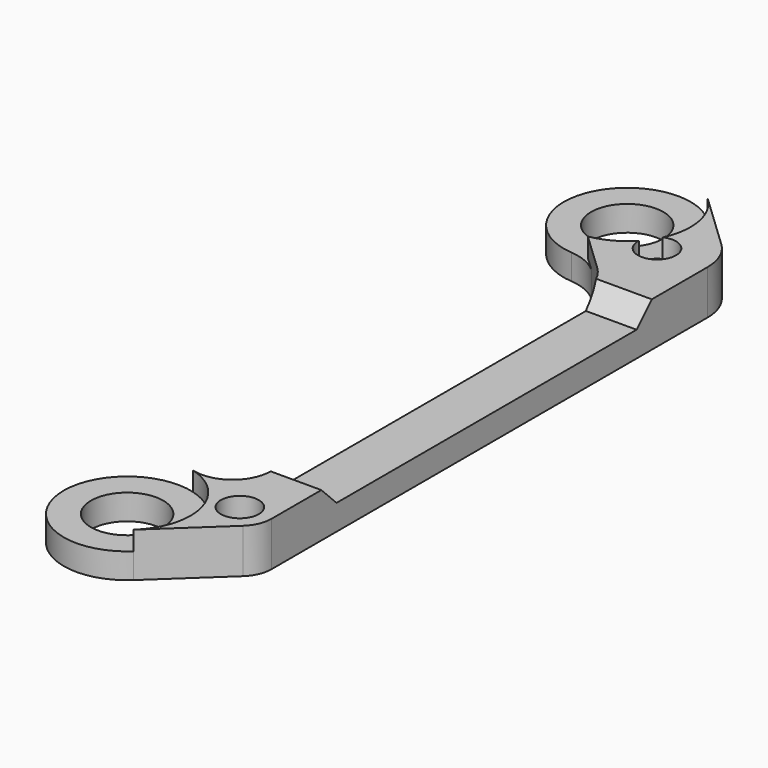
from build123d import *

# Parameters (mm, degrees)
F3_R          = 2.85
F3_R_2        = 1.5
F4_DEPTH      = 2
F5_R          = 1.5
F6_DEPTH      = 1.5
F6_DEPTH_BACK = 2
F7_SIZE       = 1.49999
F8_T1_DEPTH   = 2
F8_T6_DEPTH   = 5.7994185071
F8_T12_DEPTH  = 5.7994185071


# Not quite as in the source:
# - a fillet or chamfer that OpenCascade refuses, or shapes differently, is made with other operations: its cross-section is extruded or revolved along the edge and cut away or added
# - a fillet or chamfer is up to 0.001 mm smaller than in the source, because OpenCascade refuses the exact size


with BuildPart() as f4:
    # F3 (on Top) → F4 (new body)
    with BuildSketch(Plane.XY):
        with BuildLine():
            ThreePointArc((-19.2101191839, 28.2786664177), (-27.4339393789, 26.1039339801), (-21.8109953554, 19.7208954965))
            Line((-21.8109953554, 19.7208954965), (-17.5, 15.6341847014))
            Line((-17.5, 15.6341847014), (-17.5, -19.8340624222))
            Line((-17.5, -19.8340624222), (-18.9980046584, -21.2348967768))
            ThreePointArc((-18.9980046584, -21.2348967768), (-27.6471933185, -24.4824919767), (-19.2348967768, -28.3019953416))
            Line((-19.2348967768, -28.3019953416), (-14.2924483884, -23.6801462309))
            ThreePointArc((-14.2924483884, -23.6801462309), (-13.7066532067, -22.8494176119), (-13.5, -21.8541485601))
            Line((-13.5, -21.8541485601), (-13.5, 21.1458514399))
            ThreePointArc((-13.5, 21.1458514399), (-13.8252470415, 22.7257852025), (-14.7480953471, 24.0487845741))
            Line((-14.7480953471, 24.0487845741), (-19.2101191839, 28.2786664177))
        make_face()
        with Locations((-22.65, -24.65)):
            Circle(F3_R, mode=Mode.SUBTRACT)
        with Locations((-16, -21.8541485601)):
            Circle(F3_R_2, mode=Mode.SUBTRACT)
        with Locations((-22.65, 24.65)):
            Circle(F3_R, mode=Mode.SUBTRACT)
        with Locations((-17.5, 21.1458514399)):
            Circle(F3_R_2, mode=Mode.SUBTRACT)
    extrude(amount=F4_DEPTH)

    # F5 (on face) → F6 (join, two sides)
    with BuildSketch(Plane.XY.offset(2)) as f6_sk:
        with BuildLine():
            ThreePointArc((-18.9973102923, 21.2356394597), (-20.2798856869, 20.2474373209), (-21.8109953554, 19.7208954965))
            Line((-21.8109953554, 19.7208954965), (-17.5, 15.6341847014))
            Line((-17.5, 15.6341847014), (-13.5, 15.6341847014))
            Line((-13.5, 15.6341847014), (-13.5, 21.1458514399))
            ThreePointArc((-13.5, 21.1458514399), (-13.8252470415, 22.7257852025), (-14.7480953471, 24.0487845741))
            Line((-14.7480953471, 24.0487845741), (-19.2101191839, 28.2786664177))
            ThreePointArc((-19.2101191839, 28.2786664177), (-17.7347965939, 25.5669380986), (-18.1331588264, 22.5056712444))
            ThreePointArc((-18.1331588264, 22.5056712444), (-16.6936930608, 22.410710768), (-16, 21.1458514399))
            ThreePointArc((-16, 21.1458514399), (-17.5449141487, 19.6465240176), (-18.9973102923, 21.2356394597))
        make_face()
        with BuildLine():
            Line((-13.5, -16.9443202766), (-17.5, -16.9443202766))
            Line((-17.5, -16.9443202766), (-17.5, -19.8340624222))
            Line((-17.5, -19.8340624222), (-18.9980046584, -21.2348967768))
            ThreePointArc((-18.9980046584, -21.2348967768), (-18.9888758035, -21.2446850928), (-18.9797731837, -21.2544978108))
            ThreePointArc((-18.9797731837, -21.2544978108), (-17.6532729909, -24.8308844832), (-19.2348967768, -28.3019953416))
            Line((-19.2348967768, -28.3019953416), (-14.2924483884, -23.6801462309))
            ThreePointArc((-14.2924483884, -23.6801462309), (-13.7066532067, -22.8494176119), (-13.5, -21.8541485601))
            Line((-13.5, -21.8541485601), (-13.5, -16.9443202766))
        make_face()
        with Locations((-16, -21.8541485601)):
            Circle(F5_R, mode=Mode.SUBTRACT)
        with BuildLine():
            Line((-17.5, -19.8340624222), (-17.5, -16.9443202766))
            ThreePointArc((-17.5, -16.9443202766), (-18.6859920066, -19.3337501249), (-21.30625, -19.8339501729))
            ThreePointArc((-21.30625, -19.8339501729), (-20.0557697237, -20.3756615396), (-18.9980046584, -21.2348967768))
            Line((-18.9980046584, -21.2348967768), (-17.5, -19.8340624222))
        make_face()
    extrude(amount=F6_DEPTH)
    extrude(f6_sk.sketch, amount=-F6_DEPTH_BACK)

    # F7 (size 1.5 in the source; OpenCascade refuses exactly that, so slightly less here)
    f7_edges = [f4.edges().sort_by_distance(p)[0] for p in [
        (-15.5, -16.94432, 2),
        (-15.5, 15.634185, 2),
    ]]
    chamfer(f7_edges, length=F7_SIZE)

    # F8: fillet of radius 4 on 2 edges, made by hand

    # F8_s2 → F8_t1 (join)
    with BuildSketch(Plane.XY):
        with BuildLine():
            ThreePointArc((-17.5, 13.9144132985), (-17.8252470415, 15.4943470611), (-18.7480953471, 16.8173464327))
            Line((-18.7480953471, 16.8173464327), (-17.5, 15.6341847014))
            Line((-17.5, 15.6341847014), (-17.5, 13.9144132985))
        make_face()
        with BuildLine():
            ThreePointArc((-23.0447031853, 19.6656034071), (-21.7335895232, 19.3322992897), (-20.6085610806, 18.5810192669))
            Line((-20.6085610806, 18.5810192669), (-21.8109953554, 19.7208954965))
            ThreePointArc((-21.8109953554, 19.7208954965), (-22.4261356427, 19.6550140391), (-23.0447031853, 19.6656034071))
        make_face()
    extrude(amount=F8_T1_DEPTH)


with BuildPart() as f8_tool4:
    # F8_s5 → F8_t6 (new body)
    with BuildSketch(Plane.XY.offset(2)):
        with BuildLine():
            ThreePointArc((-17.5, 13.9144132985), (-17.8252470415, 15.4943470611), (-18.7480953471, 16.8173464327))
            Line((-18.7480953471, 16.8173464327), (-17.5, 15.6341847014))
            Line((-17.5, 15.6341847014), (-17.5, 13.9144132985))
        make_face()
    extrude(amount=F8_T6_DEPTH)

    split(bisect_by=Plane(origin=(0, 6.0670973507, -6.0670973507), x_dir=(1, 0, 0), z_dir=(0, 0.7071067812, -0.7071067812)), keep=Keep.TOP)

    split(bisect_by=Plane.XY.offset(3.5), keep=Keep.BOTTOM)


with BuildPart() as f4_1:
    add(f4.part)

    # F8_t3: union F8_tool4
    add(f8_tool4.part)


with BuildPart() as f8_tool10:
    # F8_s11 → F8_t12 (new body)
    with BuildSketch(Plane.XY.offset(2)):
        with BuildLine():
            ThreePointArc((-17.5, 13.9144132985), (-17.8252470415, 15.4943470611), (-18.7480953471, 16.8173464327))
            Line((-18.7480953471, 16.8173464327), (-17.5, 15.6341847014))
            Line((-17.5, 15.6341847014), (-17.5, 13.9144132985))
        make_face()
    extrude(amount=F8_T12_DEPTH)

    split(bisect_by=Plane.XZ.offset(-15.6341847014), keep=Keep.BOTTOM)

    split(bisect_by=Plane.XY.offset(3.5), keep=Keep.BOTTOM)


with BuildPart() as f4_2:
    add(f4_1.part)

    # F8_t9: union F8_tool10
    add(f8_tool10.part)


solid = f4_2.part
